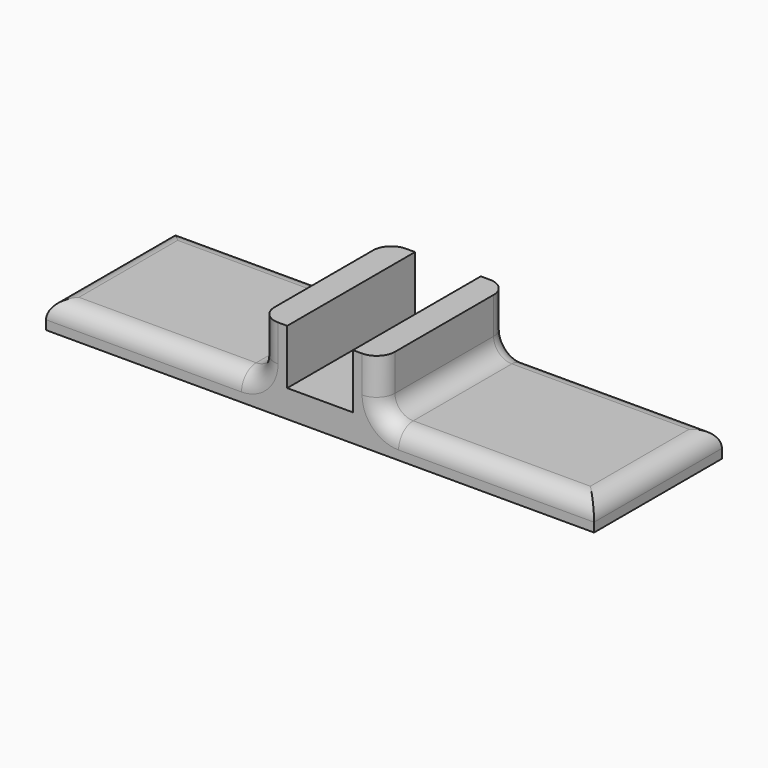
from build123d import *

# Parameters (mm, degrees)
F0_W     = 59.436
F0_H     = 44.45
F0_W_2   = 7.62
F0_W_3   = 18.288
F1_DEPTH = 7.62
F2_DEPTH = 15.24
F3_F1_R  = 5.08
F3_F2_R  = 5.08


with BuildPart() as f1:
    # F0 (on Top) → F1 (new body)
    with BuildSketch(Plane.XY):
        with Locations((-46.482, 0)):
            Rectangle(F0_W, F0_H)
        with Locations((-12.954, 0)):
            Rectangle(F0_W_2, F0_H)
        Rectangle(F0_W_3, F0_H)
        with Locations((12.954, 0)):
            Rectangle(F0_W_2, F0_H)
        with Locations((46.482, 0)):
            Rectangle(F0_W, F0_H)
    extrude(amount=-F1_DEPTH)

    # F0 (on Top) → F2 (join)
    with BuildSketch(Plane.XY):
        with Locations((-12.954, 0)):
            Rectangle(F0_W_2, F0_H)
        with Locations((12.954, 0)):
            Rectangle(F0_W_2, F0_H)
    extrude(amount=F2_DEPTH)

    # F3: fillet of radius 5.08 on 8 edges, made by hand

    # F3_f1
    f3_f1_edges = [f1.edges().sort_by_distance(p)[0] for p in [
        (16.764, 0, 0),
        (-16.764, 0, 0),
    ]]
    fillet(f3_f1_edges, radius=F3_F1_R)

    # F3_f2
    f3_f2_edges = [f1.edges().sort_by_distance(p)[0] for p in [
        (49.022, 22.225, 0),
        (76.2, 0, 0),
        (49.022, -22.225, 0),
        (-49.022, 22.225, 0),
        (-49.022, -22.225, 0),
        (-76.2, 0, 0),
        (-18.2518975516, -22.225, 1.4878975516),
        (-18.2518975516, 22.225, 1.4878975516),
        (18.2518975516, -22.225, 1.4878975516),
        (18.2518975516, 22.225, 1.4878975516),
    ]]
    fillet(f3_f2_edges, radius=F3_F2_R)


solid = f1.part
